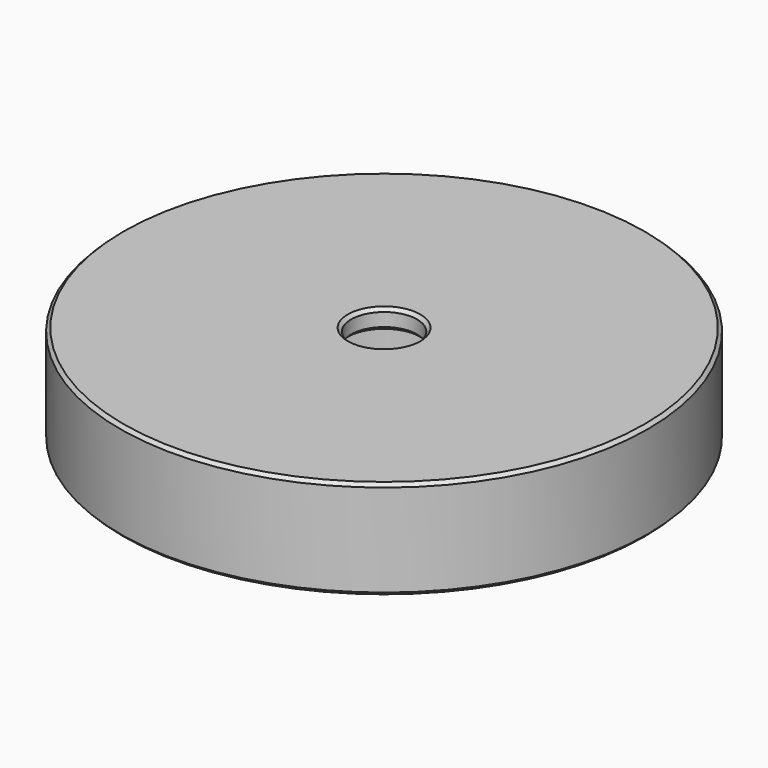
from build123d import *

# Parameters (mm, degrees)
F0_R        = 40
F0_R_2      = 5
F1_DEPTH    = 15
F4_R        = 12.5
F5_DEPTH    = 12
F6_T6_ANGLE = 90
F6_T8_ANGLE = 270


# Not quite as in the source:
# - a fillet or chamfer that OpenCascade refuses, or shapes differently, is made with other operations: its cross-section is extruded or revolved along the edge and cut away or added


with BuildPart() as f1:
    # F0 (on Top) → F1 (new body)
    with BuildSketch(Plane.XY):
        Circle(F0_R)
        Circle(F0_R_2, mode=Mode.SUBTRACT)
    extrude(amount=F1_DEPTH)

    # F2 (on Right) → F3 (revolve, cut)
    with BuildSketch(Plane.YZ):
        Polygon((-30, 0), (0, 0), (0, 5), align=None)
    revolve(axis=Axis((0, 0, -3.8595963269), (0, 0, -1)), mode=Mode.SUBTRACT)

    # F4 (on Top) → F5 (cut)
    with BuildSketch(Plane.XY):
        Circle(F4_R)
    extrude(amount=F5_DEPTH, mode=Mode.SUBTRACT)

    # F6: chamfer of 0.5 on 6 edges, made by hand

    # F6_s1 → F6_t2 (revolve, cut)
    with BuildSketch(Plane.XZ):
        Polygon((40, 14.5), (39.5, 15), (40, 15), align=None)
    revolve(axis=Axis((0, 0, 15), (0, 0, 1)), mode=Mode.SUBTRACT)

    # F6_s3 → F6_t4 (revolve, cut)
    with BuildSketch(Plane.XZ):
        Polygon((40, 0.5), (39.5, 0), (40, 0), align=None)
    revolve(axis=Axis((0, 0, 0), (0, 0, 1)), mode=Mode.SUBTRACT)

    # F6_s5 → F6_t6 (revolve, cut)
    with BuildSketch(Plane.XZ):
        Polygon((12.9178005063, 2.8470332489), (12.5, 3.3402302109), (12.5, 2.9166666667), align=None)
    revolve(axis=Axis((0, 0, 2.9166666667), (0, 0, -1)), revolution_arc=F6_T6_ANGLE, mode=Mode.SUBTRACT)

    # F6_s7 → F6_t8 (revolve, cut)
    with BuildSketch(Plane.YZ):
        Polygon((-12.9178005063, 2.8470332489), (-12.5, 3.3402302109), (-12.5, 2.9166666667), align=None)
    revolve(axis=Axis((0, 0, 2.9166666667), (0, 0, -1)), revolution_arc=F6_T8_ANGLE, mode=Mode.SUBTRACT)

    # F6_s9 → F6_t10 (revolve, cut)
    with BuildSketch(Plane.XZ):
        Polygon((5, 12.5), (5.5, 12), (5, 12), align=None)
    revolve(axis=Axis((0, 0, 12), (0, 0, -1)), mode=Mode.SUBTRACT)

    # F6_s11 → F6_t12 (revolve, cut)
    with BuildSketch(Plane.XZ):
        Polygon((5.5, 15), (5, 14.5), (5, 15), align=None)
    revolve(axis=Axis((0, 0, 15), (0, 0, 1)), mode=Mode.SUBTRACT)


solid = f1.part
